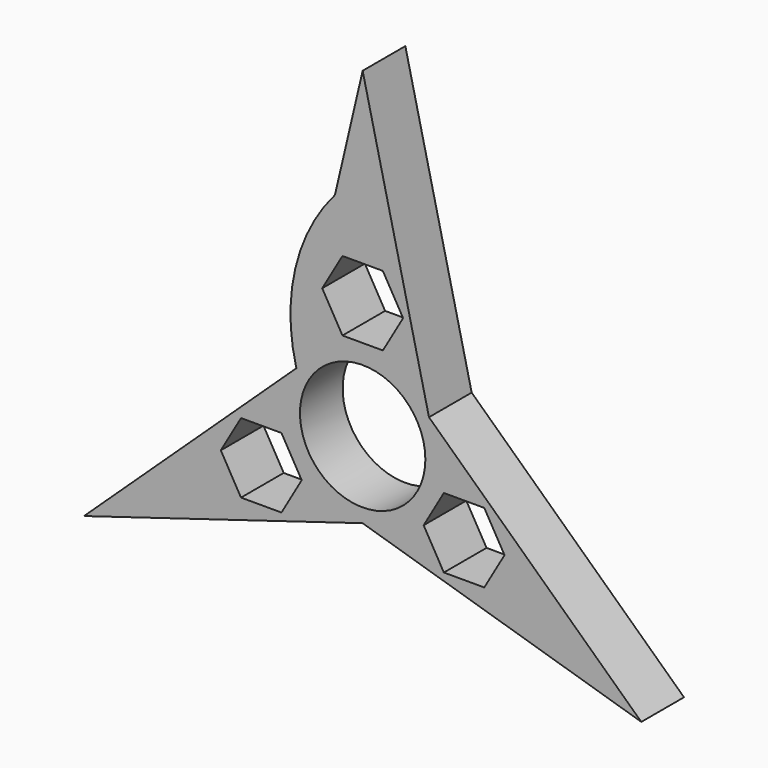
from build123d import *

# Parameters (mm, degrees)
F0_R     = 9.4
F1_DEPTH = 8
F2_DEPTH = 8


# Not quite as in the source:
# - a feature names something its author has since deleted; it is built from what else it names


with BuildPart() as f1:
    # F0 (on Front) → F1 (new body)
    with BuildSketch(Plane.XZ):
        Polygon((-4.1513990878, 30.4938093078), (-9.9419574161, 5.7399917905), (-41.7774577923, -24.1202265024), (0, -11.4799835809), (41.7774577923, -24.1202265024), (9.9419574161, 5.7399917905), (0, 48.2404530048), align=None)
        Polygon((-12.1738227533, -14.0285603702), (-18.2360010358, -14.0285603702), (-21.267090177, -8.7785599753), (-18.2360010358, -3.5285595804), (-12.1738227533, -3.5285595804), (-9.1427336121, -8.7785599753), align=None, mode=Mode.SUBTRACT)
        Polygon((18.2360010358, -3.5285595804), (21.267090177, -8.7785599753), (18.2360010358, -14.0285603702), (12.1738227533, -14.0285603702), (9.1427336121, -8.7785599753), (12.1738227533, -3.5285595804), align=None, mode=Mode.SUBTRACT)
        Circle(F0_R, mode=Mode.SUBTRACT)
        Polygon((6.0621782825, 17.5571199507), (3.0310891412, 12.3071195558), (-3.0310891412, 12.3071195558), (-6.0621782825, 17.5571199507), (-3.0310891412, 22.8071203455), (3.0310891412, 22.8071203455), align=None, mode=Mode.SUBTRACT)
    extrude(amount=F1_DEPTH)

    # F0 (on Front) → F2 (join)
    with BuildSketch(Plane.XZ):
        with BuildLine():
            ThreePointArc((-4.1513990878, 30.4938093078), (-10.107126805, 18.8328186432), (-9.9419574161, 5.7399917905))
            Line((-9.9419574161, 5.7399917905), (-4.1513990878, 30.4938093078))
        make_face()
        Polygon((-4.1513990878, 30.4938093078), (-9.9419574161, 5.7399917905), (-41.7774577923, -24.1202265024), (0, -11.4799835809), (41.7774577923, -24.1202265024), (9.9419574161, 5.7399917905), (0, 48.2404530048), align=None)
        Polygon((-12.1738227533, -14.0285603702), (-18.2360010358, -14.0285603702), (-21.267090177, -8.7785599753), (-18.2360010358, -3.5285595804), (-12.1738227533, -3.5285595804), (-9.1427336121, -8.7785599753), align=None, mode=Mode.SUBTRACT)
        Polygon((18.2360010358, -3.5285595804), (21.267090177, -8.7785599753), (18.2360010358, -14.0285603702), (12.1738227533, -14.0285603702), (9.1427336121, -8.7785599753), (12.1738227533, -3.5285595804), align=None, mode=Mode.SUBTRACT)
        Circle(F0_R, mode=Mode.SUBTRACT)
        Polygon((6.0621782825, 17.5571199507), (3.0310891412, 12.3071195558), (-3.0310891412, 12.3071195558), (-6.0621782825, 17.5571199507), (-3.0310891412, 22.8071203455), (3.0310891412, 22.8071203455), align=None, mode=Mode.SUBTRACT)
    extrude(amount=F2_DEPTH)


solid = f1.part
